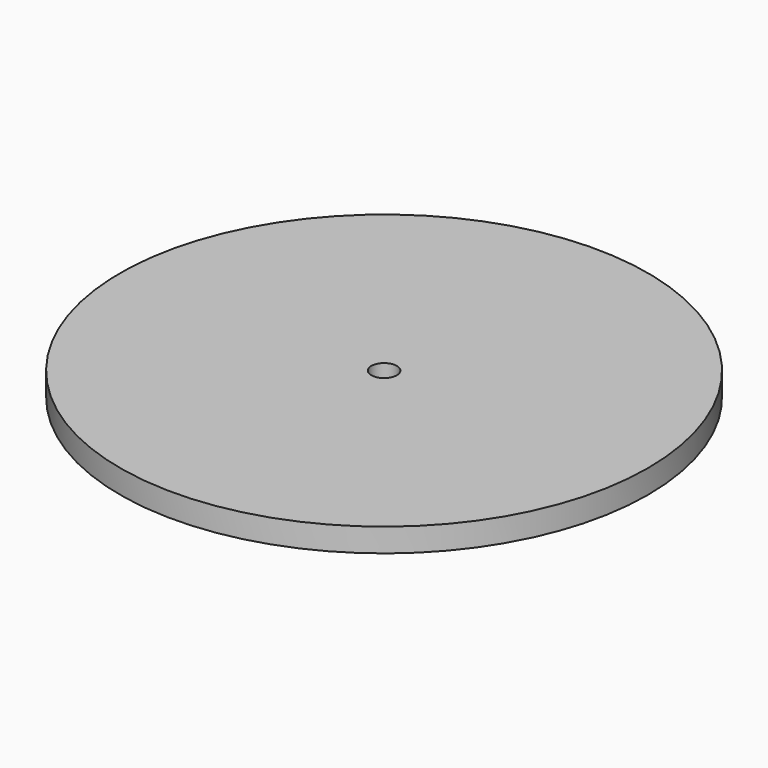
from build123d import *

# Parameters (mm, degrees)
F0_R     = 35.56
F0_R_2   = 1.7145
F1_DEPTH = 3.175
F2_DEPTH = 103


# Not quite as in the source:
# - an extrude ends at something that could not be found from the text; its depth is read off the source's solid


with BuildPart() as f1:
    # F0 (on Top) → F1 (new body)
    with BuildSketch(Plane.XY):
        Circle(F0_R)
        Circle(F0_R_2, mode=Mode.SUBTRACT)
    extrude(amount=F1_DEPTH)

    # F0 (on Top) → F2 (cut, through all)
    with BuildSketch(Plane.XY):
        Circle(F0_R)
        Circle(F0_R_2, mode=Mode.SUBTRACT)
    extrude(amount=-F2_DEPTH, mode=Mode.SUBTRACT)


solid = f1.part
